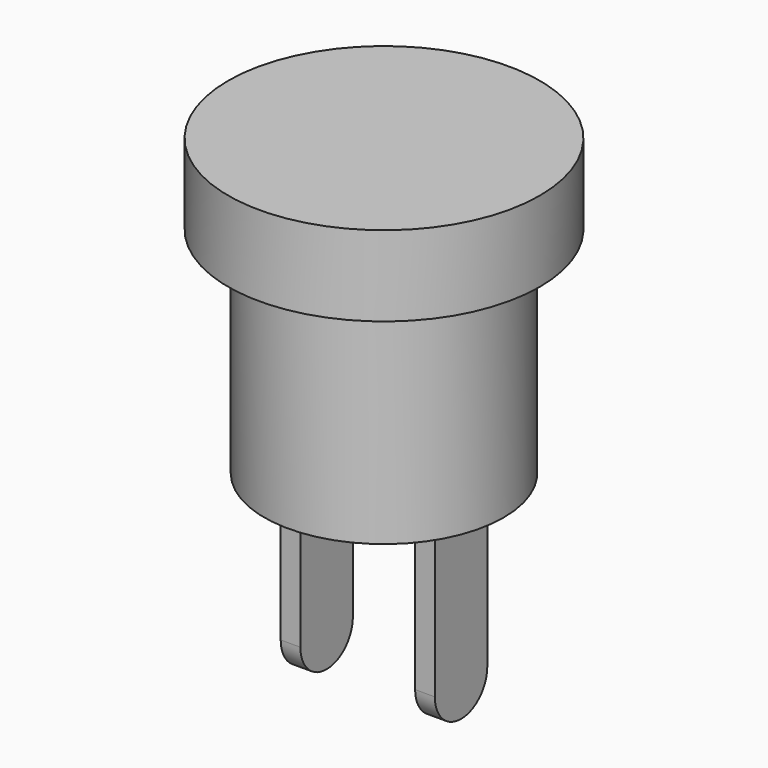
from build123d import *

# Parameters (mm, degrees)
F0_R     = 4.75
F1_DEPTH = 2.45
F2_R     = 3.65
F3_DEPTH = 6.55
F4_W     = 0.6
F4_H     = 2
F5_DEPTH = 5.83
F6_R     = 0.99999


# Not quite as in the source:
# - a fillet or chamfer is up to 0.001 mm smaller than in the source, because OpenCascade refuses the exact size


with BuildPart() as f1:
    # F0 (on Top) → F1 (new body)
    with BuildSketch(Plane.XY):
        Circle(F0_R)
    extrude(amount=-F1_DEPTH)

    # F2 (on face) → F3 (join)
    with BuildSketch(Plane(origin=(0, 0, -2.45), x_dir=(1, 0, 0), z_dir=(0, 0, -1))):
        Circle(F2_R)
    extrude(amount=F3_DEPTH)

    # F4 (on face) → F5 (join)
    with BuildSketch(Plane(origin=(0, 0, -9), x_dir=(1, 0, 0), z_dir=(0, 0, -1))):
        with Locations((-2.05, 0)):
            Rectangle(F4_W, F4_H)
        with Locations((2.05, 0)):
            Rectangle(F4_W, F4_H)
    extrude(amount=F5_DEPTH)

    # F6 (radius 1 in the source; OpenCascade refuses exactly that, so slightly less here)
    f6_edges = [f1.edges().sort_by_distance(p)[0] for p in [
        (-2.05, -1, -14.83),
        (2.05, -1, -14.83),
        (2.05, 1, -14.83),
        (-2.05, 1, -14.83),
    ]]
    fillet(f6_edges, radius=F6_R)


solid = f1.part
